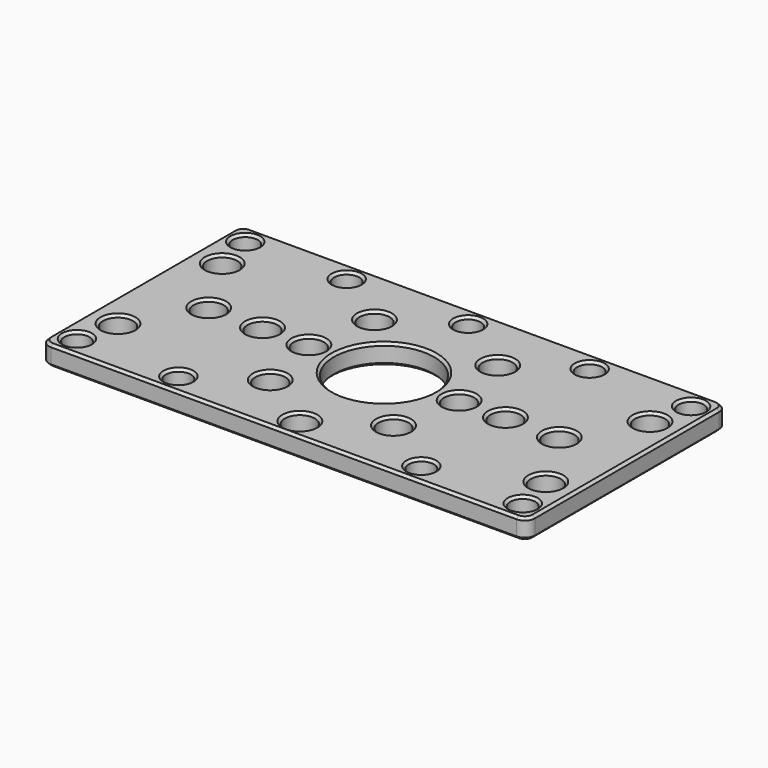
from build123d import *

# Parameters (mm, degrees)
F0_W     = 97
F0_H     = 50
F0_R     = 2.5
F0_R_2   = 3
F0_R_3   = 10
F1_DEPTH = 4
F2_R     = 2
F3_SIZE  = 0.49999


# Not quite as in the source:
# - a fillet or chamfer is up to 0.001 mm smaller than in the source, because OpenCascade refuses the exact size


with BuildPart() as f1:
    # F0 (on Top) → F1 (new body)
    with BuildSketch(Plane.XY):
        Rectangle(F0_W, F0_H)
        with Locations((-44.5, -21)):
            Circle(F0_R, mode=Mode.SUBTRACT)
        with Locations((-42.7, -13)):
            Circle(F0_R_2, mode=Mode.SUBTRACT)
        with Locations((-24.25, -21)):
            Circle(F0_R, mode=Mode.SUBTRACT)
        with Locations((-12.3, -13)):
            Circle(F0_R_2, mode=Mode.SUBTRACT)
        with Locations((0, -21)):
            Circle(F0_R_2, mode=Mode.SUBTRACT)
        with Locations((12.3, -13)):
            Circle(F0_R_2, mode=Mode.SUBTRACT)
        with Locations((24.25, -21)):
            Circle(F0_R, mode=Mode.SUBTRACT)
        with Locations((44.5, -21)):
            Circle(F0_R, mode=Mode.SUBTRACT)
        with Locations((42.7, -13)):
            Circle(F0_R_2, mode=Mode.SUBTRACT)
        with Locations((-35, 0)):
            Circle(F0_R_2, mode=Mode.SUBTRACT)
        with Locations((-24.25, 0)):
            Circle(F0_R_2, mode=Mode.SUBTRACT)
        with Locations((-15, 0)):
            Circle(F0_R_2, mode=Mode.SUBTRACT)
        with Locations((-42.7, 13)):
            Circle(F0_R_2, mode=Mode.SUBTRACT)
        with Locations((-44.5, 21)):
            Circle(F0_R, mode=Mode.SUBTRACT)
        with Locations((-12.3, 13)):
            Circle(F0_R_2, mode=Mode.SUBTRACT)
        with Locations((-24.25, 21)):
            Circle(F0_R, mode=Mode.SUBTRACT)
        Circle(F0_R_3, mode=Mode.SUBTRACT)
        with Locations((15, 0)):
            Circle(F0_R_2, mode=Mode.SUBTRACT)
        with Locations((24.25, 0)):
            Circle(F0_R_2, mode=Mode.SUBTRACT)
        with Locations((35, 0)):
            Circle(F0_R_2, mode=Mode.SUBTRACT)
        with Locations((12.3, 13)):
            Circle(F0_R_2, mode=Mode.SUBTRACT)
        with Locations((0, 21)):
            Circle(F0_R, mode=Mode.SUBTRACT)
        with Locations((42.7, 13)):
            Circle(F0_R_2, mode=Mode.SUBTRACT)
        with Locations((24.25, 21)):
            Circle(F0_R, mode=Mode.SUBTRACT)
        with Locations((44.5, 21)):
            Circle(F0_R, mode=Mode.SUBTRACT)
    extrude(amount=F1_DEPTH)

    # F2
    f2_edges = [f1.edges().sort_by_distance(p)[0] for p in [
        (-48.5, 25, 2),
        (-48.5, -25, 2),
        (48.5, -25, 2),
        (48.5, 25, 2),
    ]]
    fillet(f2_edges, radius=F2_R)

    # F3 (size 0.5 in the source; OpenCascade refuses exactly that, so slightly less here)
    f3_edges = [f1.edges().sort_by_distance(p)[0] for p in [
        (0, -25, 4),
        (-47.914214, -24.414214, 4),
        (47.914214, -24.414214, 4),
        (-48.5, 0, 4),
        (48.5, 0, 4),
        (-47.914214, 24.414214, 4),
        (47.914214, 24.414214, 4),
        (0, 25, 4),
        (-47, -21, 4),
        (-45.7, -13, 4),
        (-26.75, -21, 4),
        (-15.3, -13, 4),
        (-3, -21, 4),
        (9.3, -13, 4),
        (21.75, -21, 4),
        (42, -21, 4),
        (39.7, -13, 4),
        (-38, 0, 4),
        (-27.25, 0, 4),
        (-18, 0, 4),
        (-45.7, 13, 4),
        (-47, 21, 4),
        (-15.3, 13, 4),
        (-26.75, 21, 4),
        (-10, 0, 4),
        (12, 0, 4),
        (21.25, 0, 4),
        (32, 0, 4),
        (9.3, 13, 4),
        (-2.5, 21, 4),
        (39.7, 13, 4),
        (21.75, 21, 4),
        (42, 21, 4),
        (0, -25, 0),
        (-47.914214, -24.414214, 0),
        (47.914214, -24.414214, 0),
        (-48.5, 0, 0),
        (48.5, 0, 0),
        (-47.914214, 24.414214, 0),
        (47.914214, 24.414214, 0),
        (0, 25, 0),
        (-47, -21, 0),
        (-45.7, -13, 0),
        (-26.75, -21, 0),
        (-15.3, -13, 0),
        (-3, -21, 0),
        (9.3, -13, 0),
        (21.75, -21, 0),
        (42, -21, 0),
        (39.7, -13, 0),
        (-38, 0, 0),
        (-27.25, 0, 0),
        (-18, 0, 0),
        (-45.7, 13, 0),
        (-47, 21, 0),
        (-15.3, 13, 0),
        (-26.75, 21, 0),
        (-10, 0, 0),
        (12, 0, 0),
        (21.25, 0, 0),
        (32, 0, 0),
        (9.3, 13, 0),
        (-2.5, 21, 0),
        (39.7, 13, 0),
        (21.75, 21, 0),
        (42, 21, 0),
    ]]
    chamfer(f3_edges, length=F3_SIZE)


solid = f1.part
